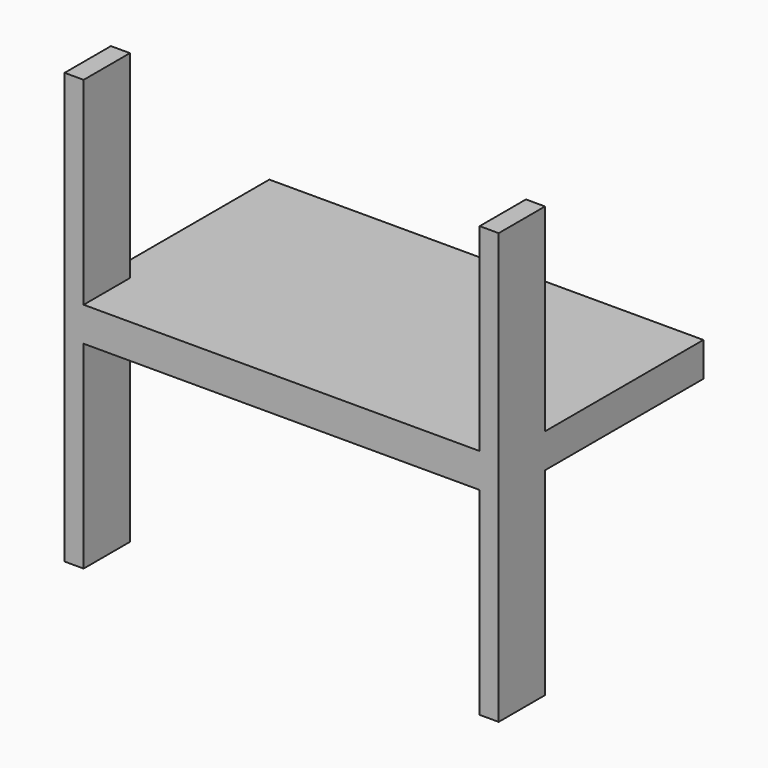
from build123d import *

# Parameters (mm, degrees)
F2_DEPTH = 1320.8
F1_W     = 127
F1_H     = 1320.8
F3_DEPTH = 386.08


# Not quite as in the source:
# - a feature names something its author has since deleted; it is built from what else it names


with BuildPart() as f2:
    # F1 (on Front) → F2 (new body)
    with BuildSketch(Plane.XZ):
        Polygon((-543.1821789121, 381.5627378464), (-670.1821789121, 381.5627378464), (-670.1821789121, 152.9627378464), (-543.1821789121, 152.9627378464), (2098.4178210879, 152.9627378464), (2225.4178210879, 152.9627378464), (2225.4178210879, 381.5627378464), (2098.4178210879, 381.5627378464), align=None)
    extrude(amount=-F2_DEPTH)

    # F1 (on Front) → F3 (join)
    with BuildSketch(Plane.XZ):
        with Locations((-606.6821789121, 1041.9627378464)):
            Rectangle(F1_W, F1_H)
        Polygon((-543.1821789121, 381.5627378464), (-670.1821789121, 381.5627378464), (-670.1821789121, 152.9627378464), (-543.1821789121, 152.9627378464), (2098.4178210879, 152.9627378464), (2225.4178210879, 152.9627378464), (2225.4178210879, 381.5627378464), (2098.4178210879, 381.5627378464), align=None)
        with Locations((-606.6821789121, -507.4372621536)):
            Rectangle(F1_W, F1_H)
        with Locations((2161.9178210879, 1041.9627378464)):
            Rectangle(F1_W, F1_H)
        with Locations((2161.9178210879, -507.4372621536)):
            Rectangle(F1_W, F1_H)
    extrude(amount=F3_DEPTH)


solid = f2.part
